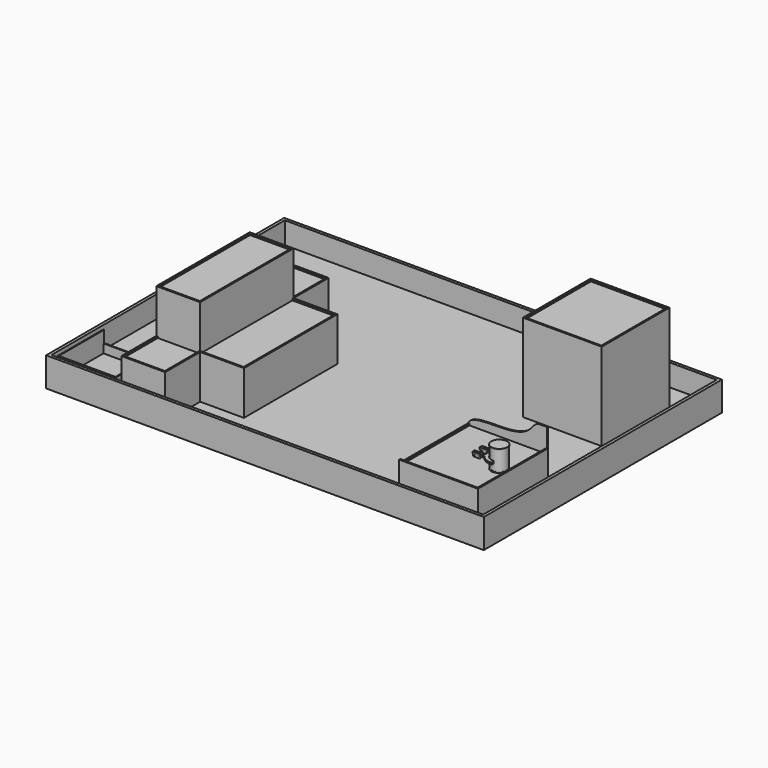
from build123d import *

# Parameters (mm, degrees)
F0_R      = 27.2
F1_DEPTH  = 2.83
F2_R      = 26.4
F3_DEPTH  = 67.36
F4_R      = 27.2
F5_DEPTH  = 2.83
F9_W      = 270
F9_H      = 300
F10_DEPTH = 72
F12_DEPTH = 15
F14_DEPTH = 5
F15_W     = 5
F15_H     = 290
F16_DEPTH = 5
F17_W     = 1500
F17_H     = 1020
F18_DEPTH = 25
F19_W     = 270
F19_H     = 290
F20_DEPTH = 300
F21_W     = 260
F21_H     = 280
F22_DEPTH = 5
F23_W     = 1500
F23_H     = 1020
F23_W_2   = 1480
F23_H_2   = 1000
F24_DEPTH = 75
F26_DEPTH = 150
F27_W     = 150
F27_H     = 400
F28_DEPTH = 150
F29_W     = 140
F29_H     = 390
F30_DEPTH = 5
F31_W     = 140
F31_H     = 145
F31_W_2   = 145
F31_H_2   = 390
F32_DEPTH = 5
F33_R     = 3
F34_DEPTH = 4
F35_R     = 3.99999
F35_2_R   = 3.99999
F36_R     = 3
F37_DEPTH = 8
F38_R     = 3
F39_DEPTH = 8
F40_R     = 3
F40_R_2   = 2.5
F41_DEPTH = 3
F42_R     = 3
F42_R_2   = 2.5
F43_DEPTH = 3
F45_DEPTH = 270.001
F46_W     = 200
F46_H     = 200
F46_W_2   = 194
F46_H_2   = 191
F47_DEPTH = 30
F49_DEPTH = 40
F50_R     = 2.6355555969
F50_R_2   = 2.5249535516
F50_R_3   = 2.6788042429
F50_R_4   = 2.7425777
F51_DEPTH = 6


# Not quite as in the source:
# - a fillet or chamfer is up to 0.001 mm smaller than in the source, because OpenCascade refuses the exact size
# - a feature names something its author has since deleted; it is built from what else it names


with BuildPart() as f1:
    # F0 (on Top) → F1 (new body)
    with BuildSketch(Plane.XY):
        Circle(F0_R)
    extrude(amount=F1_DEPTH)

    # F2 (on face) → F3 (join)
    with BuildSketch(Plane.XY.offset(2.83)):
        Circle(F2_R)
    extrude(amount=F3_DEPTH)

    # F4 (on face) → F5 (join)
    with BuildSketch(Plane.XY.offset(70.19)):
        Circle(F4_R)
    extrude(amount=F5_DEPTH)


with BuildPart() as f10:
    # F9 (on Top) → F10 (new body)
    with BuildSketch(Plane.XY):
        with Locations((-87.8, 0)):
            Rectangle(F9_W, F9_H)
    extrude(amount=-F10_DEPTH)

    # F11 (on face) → F12 (join)
    with BuildSketch(Plane.XY):
        Polygon((-222.8, -145), (-222.8, -150), (47.2, -150), (47.2, 150), (42.2, 150), (42.2, -145), align=None)
    extrude(amount=F12_DEPTH)

    # F13 (on face) → F14 (join)
    with BuildSketch(Plane(origin=(0, 150, 0), x_dir=(-1, 0, 0), z_dir=(0, 1, 0))):
        with BuildLine():
            Line((-21.3134280931, 81.3575685024), (-47.2, 81.3575685024))
            Line((-47.2, 81.3575685024), (-47.2, -72))
            Line((-47.2, -72), (222.8, -72))
            Line((222.8, -72), (222.8, 0))
            add(Edge.make_bspline(
                [(-21.3134280931, 81.3575685024), (-6.3059147253, 81.3822787863), (12.9585432644, 38.1268753575), (103.6097013063, 23.6068887567), (223.0224295336, 30.7718731823), (222.8, 0)],
                knots=[0, 0, 0, 0, 0.2487100673, 0.6151112321, 1, 1, 1, 1], degree=3))
        make_face()
    extrude(amount=-F14_DEPTH)

    # F15 (on face) → F16 (join)
    with BuildSketch(Plane.XY):
        with Locations((-220.3, 0)):
            Rectangle(F15_W, F15_H)
    extrude(amount=F16_DEPTH)

    # F17 (on face) → F18 (join)
    with BuildSketch(Plane(origin=(0, 0, -72), x_dir=(1, 0, 0), z_dir=(0, 0, -1))):
        with Locations((-602.8, -260)):
            Rectangle(F17_W, F17_H)
    extrude(amount=F18_DEPTH)

    # F19 (on face) → F20 (join)
    with BuildSketch(Plane.XY.offset(-72)):
        with Locations((-87.8, 525)):
            Rectangle(F19_W, F19_H)
    extrude(amount=F20_DEPTH)

    # F21 (on face) → F22 (cut)
    with BuildSketch(Plane.XY.offset(228)):
        with Locations((-87.8, 525)):
            Rectangle(F21_W, F21_H)
    extrude(amount=-F22_DEPTH, mode=Mode.SUBTRACT)

    # F23 (on face) → F24 (join)
    with BuildSketch(Plane.XY.offset(-72)):
        with Locations((-602.8, 260)):
            Rectangle(F23_W, F23_H)
        with Locations((-602.8, 260)):
            Rectangle(F23_W_2, F23_H_2, mode=Mode.SUBTRACT)
    extrude(amount=F24_DEPTH)

    # F25 (on face) → F26 (join)
    with BuildSketch(Plane.XY.offset(-72)):
        Polygon((-952.8, 460), (-1102.8, 460), (-1102.8, -240), (-952.8, -240), (-952.8, -90), (-802.8, -90), (-802.8, 310), (-952.8, 310), align=None)
    extrude(amount=F26_DEPTH)

    # F27 (on face) → F28 (join)
    with BuildSketch(Plane.XY.offset(78)):
        with Locations((-1027.8, 110)):
            Rectangle(F27_W, F27_H)
    extrude(amount=F28_DEPTH)

    # F29 (on face) → F30 (cut)
    with BuildSketch(Plane.XY.offset(228)):
        with Locations((-1027.8, 110)):
            Rectangle(F29_W, F29_H)
    extrude(amount=-F30_DEPTH, mode=Mode.SUBTRACT)

    # F31 (on face) → F32 (cut)
    with BuildSketch(Plane.XY.offset(78)):
        with Locations((-1027.8, 382.5)):
            Rectangle(F31_W, F31_H)
        with Locations((-880.3, 110)):
            Rectangle(F31_W_2, F31_H_2)
        with Locations((-1027.8, -162.5)):
            Rectangle(F31_W, F31_H)
    extrude(amount=-F32_DEPTH, mode=Mode.SUBTRACT)

    # F46 (on face) → F47 (join)
    with BuildSketch(Plane.XY.offset(-72)):
        with Locations((-1232.8, -130)):
            Rectangle(F46_W, F46_H)
        with Locations((-1232.8, -128.5)):
            Rectangle(F46_W_2, F46_H_2, mode=Mode.SUBTRACT)
    extrude(amount=F47_DEPTH)

    # F48 (on face) → F49 (join)
    with BuildSketch(Plane.XY.offset(-42)):
        Polygon((-1329.8, -30), (-1332.8, -30), (-1332.8, -230), (-1329.8, -230), (-1135.8, -230), (-1132.8, -230), (-1132.8, -30), (-1135.8, -30), (-1135.8, -224), (-1329.8, -224), align=None)
    extrude(amount=F49_DEPTH)


with BuildPart() as f34:
    # F33 (on offset) → F34 (new body, symmetric)
    with BuildSketch(Plane.XY.offset(25)):
        with BuildLine():
            Line((-55, -12), (-74.5, -12))
            Line((-74.5, -12), (-74.5, -13))
            Line((-74.5, -13), (-65.6457513111, -13))
            ThreePointArc((-65.6457513111, -13), (-67, -16), (-65.6457513111, -19))
            Line((-65.6457513111, -19), (-74.5, -19))
            Line((-74.5, -19), (-74.5, -20))
            Line((-74.5, -20), (-55, -20))
            ThreePointArc((-55, -20), (-51, -16), (-55, -12))
        make_face()
        with Locations((-63, -16)):
            Circle(F33_R, mode=Mode.SUBTRACT)
        with Locations((-55, -16)):
            Circle(F33_R, mode=Mode.SUBTRACT)
    extrude(amount=F34_DEPTH, both=True)

    # F35 (radius 4 in the source; OpenCascade refuses exactly that, so slightly less here)
    f35_edges = [f34.edges().sort_by_distance(p)[0] for p in [
        (-74.5, -19.5, 29),
        (-74.5, -12.5, 29),
        (-74.5, -19.5, 21),
        (-74.5, -12.5, 21),
    ]]
    fillet(f35_edges, radius=F35_R)

    # F36 (on face) → F37 (join, through all)
    with BuildSketch(Plane.XZ.offset(20)):
        with Locations((-70.5, 25)):
            Circle(F36_R)
    extrude(amount=-F37_DEPTH)

    # F42 (on offset) → F43 (join, symmetric)
    with BuildSketch(Plane.XY.offset(25)):
        with Locations((-63, -16)):
            Circle(F42_R)
        with Locations((-63, -16)):
            Circle(F42_R_2, mode=Mode.SUBTRACT)
        with Locations((-55, -16)):
            Circle(F42_R)
        with Locations((-55, -16)):
            Circle(F42_R_2, mode=Mode.SUBTRACT)
    extrude(amount=F43_DEPTH, both=True)


with BuildPart() as f34b:
    # F33 (on offset) → F34, piece 2 (new body, symmetric)
    with BuildSketch(Plane.XY.offset(25)):
        with BuildLine():
            Line((-74.5, 13), (-74.5, 12))
            Line((-74.5, 12), (-55, 12))
            ThreePointArc((-55, 12), (-51, 16), (-55, 20))
            Line((-55, 20), (-74.5, 20))
            Line((-74.5, 20), (-74.5, 19))
            Line((-74.5, 19), (-65.6457513111, 19))
            ThreePointArc((-65.6457513111, 19), (-67, 16), (-65.6457513111, 13))
            Line((-65.6457513111, 13), (-74.5, 13))
        make_face()
        with Locations((-63, 16)):
            Circle(F33_R, mode=Mode.SUBTRACT)
        with Locations((-55, 16)):
            Circle(F33_R, mode=Mode.SUBTRACT)
    extrude(amount=F34_DEPTH, both=True)

    # F35#2 (radius 4 in the source; OpenCascade refuses exactly that, so slightly less here)
    f35_2_edges = [f34b.edges().sort_by_distance(p)[0] for p in [
        (-74.5, 12.5, 29),
        (-74.5, 19.5, 29),
        (-74.5, 19.5, 21),
        (-74.5, 12.5, 21),
    ]]
    fillet(f35_2_edges, radius=F35_2_R)

    # F38 (on face) → F39 (join, through all)
    with BuildSketch(Plane(origin=(0, 20, 0), x_dir=(-1, 0, 0), z_dir=(0, 1, 0))):
        with Locations((70.5, 25)):
            Circle(F38_R)
    extrude(amount=-F39_DEPTH)

    # F40 (on offset) → F41 (join, symmetric)
    with BuildSketch(Plane.XY.offset(25)):
        with Locations((-55, 16)):
            Circle(F40_R)
        with Locations((-55, 16)):
            Circle(F40_R_2, mode=Mode.SUBTRACT)
        with Locations((-63, 16)):
            Circle(F40_R)
        with Locations((-63, 16)):
            Circle(F40_R_2, mode=Mode.SUBTRACT)
    extrude(amount=F41_DEPTH, both=True)


with BuildPart() as f45_tool:
    # F44 (on face) → F45 (new body, through all)
    with BuildSketch(Plane(origin=(0, 20, 0), x_dir=(-1, 0, 0), z_dir=(0, 1, 0))):
        with BuildLine():
            Line((71.5, 26), (71.5, 27.2912878475))
            ThreePointArc((71.5, 27.2912878475), (70.5, 27.5), (69.5, 27.2912878475))
            Line((69.5, 27.2912878475), (69.5, 26))
            Line((69.5, 26), (68.2087121525, 26))
            ThreePointArc((68.2087121525, 26), (68, 25), (68.2087121525, 24))
            Line((68.2087121525, 24), (69.5, 24))
            Line((69.5, 24), (69.5, 22.7087121525))
            ThreePointArc((69.5, 22.7087121525), (70.5, 22.5), (71.5, 22.7087121525))
            Line((71.5, 22.7087121525), (71.5, 24))
            Line((71.5, 24), (72.7912878475, 24))
            ThreePointArc((72.7912878475, 24), (73, 25), (72.7912878475, 26))
            Line((72.7912878475, 26), (71.5, 26))
        make_face()
    extrude(amount=-F45_DEPTH)


with BuildPart() as f34_1:
    add(f34.part)

    # F45: cut by f45_tool
    add(f45_tool.part, mode=Mode.SUBTRACT)


with BuildPart() as f34b_1:
    add(f34b.part)

    # F45: cut by f45_tool
    add(f45_tool.part, mode=Mode.SUBTRACT)


with BuildPart() as f51:
    # F50 (on face) → F51 (new body)
    with BuildSketch(Plane.XY.offset(29)):
        with BuildLine():
            Line((-33.2819414696, 21.0185684264), (-75.7019817829, 21.0185684264))
            Line((-75.7019817829, 21.0185684264), (-75.7019817829, 10.6598846614))
            Line((-75.7019817829, 10.6598846614), (-37.7754436599, 10.6598846614))
            ThreePointArc((-37.7754436599, 10.6598846614), (-39.1643948243, -0.414831189), (-37.40703767, -11.4370910451))
            Line((-37.40703767, -11.4370910451), (-75.3002762794, -11.4370910451))
            Line((-75.3002762794, -11.4370910451), (-75.3002762794, -20.7782350481))
            Line((-75.3002762794, -20.7782350481), (-33.1266104634, -20.7782350481))
            ThreePointArc((-33.1266104634, -20.7782350481), (-18.7391213167, -34.3998945699), (0.446818726, -39.3445034273))
            ThreePointArc((0.446818726, -39.3445034273), (6.064294, -33.3406599861), (0.4386114015, -27.3445062339))
            ThreePointArc((0.4386114015, -27.3445062339), (-27.1676177227, -0.1094223507), (-0.2704305516, 27.8261285275))
            ThreePointArc((-0.2704305516, 27.8261285275), (3.9820059197, 33.9344174365), (-0.5706181242, 39.8223732492))
            ThreePointArc((-0.5706181242, 39.8223732492), (-19.3104440822, 34.5679914901), (-33.2819414696, 21.0185684264))
        make_face()
        with Locations((-63, -16)):
            Circle(F50_R, mode=Mode.SUBTRACT)
        with Locations((-55.0504773855, -16.0028897226)):
            Circle(F50_R_2, mode=Mode.SUBTRACT)
        with Locations((-63, 16)):
            Circle(F50_R_3, mode=Mode.SUBTRACT)
        with Locations((-55, 16)):
            Circle(F50_R_4, mode=Mode.SUBTRACT)
    extrude(amount=F51_DEPTH)


solid = Compound([f1.part, f10.part, f34_1.part, f34b_1.part, f51.part])
